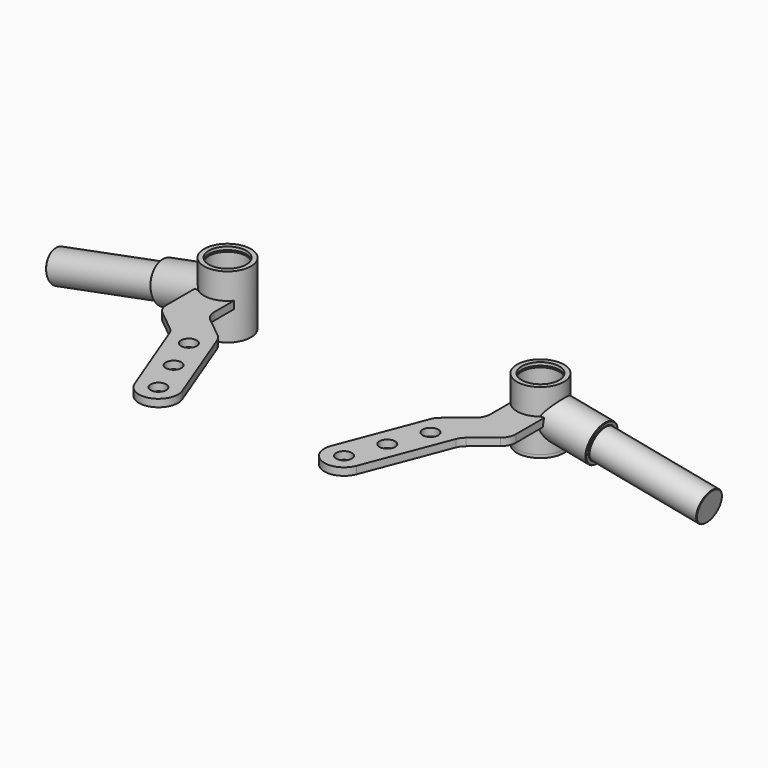
from build123d import *

# Parameters (mm, degrees)
F0_R      = 15
F0_R_2    = 12
F1_DEPTH  = 19
F2_R      = 15
F2_R_2    = 10.5
F3_DEPTH  = 2
F4_W      = 2
F4_H      = 1
F7_R      = 10
F8_DEPTH  = 70
F10_ANGLE = -11
F11_R     = 12.5
F12_REACH = 93.7061177232
F13_SIZE  = 0.3
F14_R     = 5
F15_DEPTH = 2.4
F16_R     = 10


with BuildPart() as f1:
    # F0 (on Top) → F1 (new body, symmetric)
    with BuildSketch(Plane.XY):
        Circle(F0_R)
        Circle(F0_R_2, mode=Mode.SUBTRACT)
    extrude(amount=F1_DEPTH, both=True)

    # F2 (on face) → F3 (join)
    with BuildSketch(Plane(origin=(0, 0, -19), x_dir=(1, 0, 0), z_dir=(0, 0, -1))):
        Circle(F2_R)
        Circle(F2_R_2, mode=Mode.SUBTRACT)
    extrude(amount=F3_DEPTH)

    # F4 (on Front) → F5 (revolve, cut)
    with BuildSketch(Plane.XZ):
        with Locations((12, 16.5)):
            Rectangle(F4_W, F4_H)
    revolve(axis=Axis((0, 0, 8.6649929517), (0, 0, 1)), mode=Mode.SUBTRACT)


with BuildPart() as f8:
    # F7 (on offset) → F8 (new body)
    with BuildSketch(Plane.YZ.offset(40)):
        Circle(F7_R)
    extrude(amount=F8_DEPTH)


with BuildPart() as f8_1:
    # F10: moved
    add(f8.part.rotate(Axis((0, -48.5732145607, 0), (0, -1, 0)), F10_ANGLE))

    f12_end = f1.part.faces().sort_by_distance((-15, 0, -1))[0]
    # F11 (on face) → F12 (join, up to a face of F1 that its end follows)
    with BuildSketch(Plane(origin=(39.2650873379, 0, -7.6323598151), x_dir=(0, -1, 0), z_dir=(-0.9816271834, 0, 0.1908089954))):
        Circle(F11_R)
    f12_long = extrude(amount=F12_REACH, mode=Mode.PRIVATE)
    add(split(f12_long, bisect_by=f12_end, keep=Keep.ALL, mode=Mode.PRIVATE).solids().sort_by_distance((39.2650873379, 0, -7.6323598151))[0])

    # F13
    f13_edges = [f8_1.edges().sort_by_distance(p)[0] for p in [
        (39.265087, -10, -7.63236),
        (107.97899, -10, -20.988989),
        (39.265087, 12.5, -7.63236),
    ]]
    chamfer(f13_edges, length=F13_SIZE)


with BuildPart() as f15:
    # F14 (on Top) → F15 (new body, symmetric)
    with BuildSketch(Plane.XY):
        with BuildLine():
            Line((-30.875182133, -45.5522479748), (-52.3772591057, -101.5670735646))
            ThreePointArc((-52.3772591057, -101.5670735646), (-45.1871031438, -117.7164282651), (-29.0377484433, -110.5262723032))
            Line((-29.0377484433, -110.5262723032), (-7.5356714706, -54.5114467134))
            Line((-7.5356714706, -54.5114467134), (11.6697553312, -38.9591987386))
            Line((11.6697553312, -38.9591987386), (11.6697553312, -9.4242671073))
            ThreePointArc((11.6697553312, -9.4242671073), (0, -15), (-11.6697553312, -9.4242671073))
            Line((-11.6697553312, -9.4242671073), (-11.6697553312, -30))
            Line((-11.6697553312, -30), (-30.875182133, -45.5522479748))
        make_face()
        with Locations((-40.7075037745, -106.0466729339)):
            Circle(F14_R, mode=Mode.SUBTRACT)
        with Locations((-31.7483050359, -82.7071622715)):
            Circle(F14_R, mode=Mode.SUBTRACT)
        with Locations((-22.7891062972, -59.3676516091)):
            Circle(F14_R, mode=Mode.SUBTRACT)
    extrude(amount=F15_DEPTH, both=True)

    # F16
    f16_edges = [f15.edges().sort_by_distance(p)[0] for p in [
        (-7.535671, -54.511447, 0),
        (11.669755, -38.959199, 0),
        (-30.875182, -45.552248, 0),
        (-11.669755, -30, 0),
    ]]
    fillet(f16_edges, radius=F16_R)


with BuildPart() as f18_1:
    # F18: instance of F8
    add(f8_1.part.mirror(Plane.YZ.offset(-100)))


with BuildPart() as f18_2:
    # F18: instance of F1
    add(f1.part.mirror(Plane.YZ.offset(-100)))


with BuildPart() as f18_3:
    # F18: instance of F15
    add(f15.part.mirror(Plane.YZ.offset(-100)))


solid = Compound([f1.part, f8_1.part, f15.part, f18_1.part, f18_2.part, f18_3.part])
